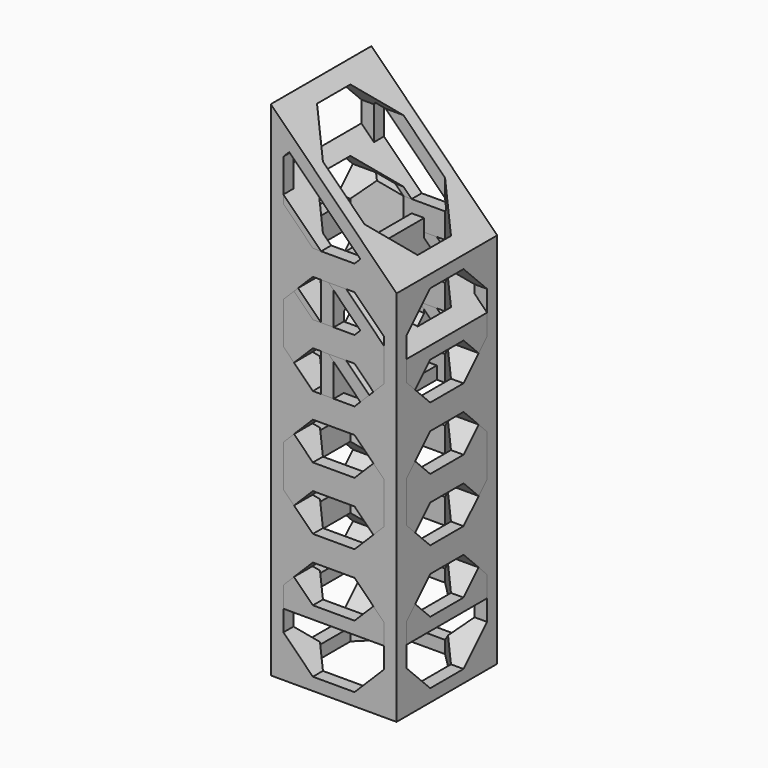
from build123d import *

# Parameters (mm, degrees)
F0_W      = 10
F0_H      = 10
F1_DEPTH  = 5
F3_DEPTH  = 10
F5_DEPTH  = 10
F7_DEPTH  = 10
F8_W      = 10
F8_H      = 20
F9_DEPTH  = 5
F11_DEPTH = 10
F13_DEPTH = 10
F15_DEPTH = 20
F17_DEPTH = 5
F19_DEPTH = 10
F21_DEPTH = 10
F23_DEPTH = 15
F25_DEPTH = 5
F27_DEPTH = 5
F29_DEPTH = 10
F31_DEPTH = 10
F33_DEPTH = 20
F35_DEPTH = 5
F37_DEPTH = 10
F39_DEPTH = 10
F41_DEPTH = 30
F43_DEPTH = 5
F45_DEPTH = 10
F47_DEPTH = 10
F49_DEPTH = 40


with BuildPart() as f1:
    # F0 (on Front) → F1 (new body, symmetric)
    with BuildSketch(Plane.XZ):
        Rectangle(F0_W, F0_H)
    extrude(amount=F1_DEPTH, both=True)

    # F2 (on face) → F3 (cut, through all)
    with BuildSketch(Plane.XZ.offset(5)):
        Polygon((4, 1.6568542495), (1.6568542495, 4), (-1.6568542495, 4), (-4, 1.6568542495), (-4, -1.6568542495), (-1.6568542495, -4), (1.6568542495, -4), (4, -1.6568542495), align=None)
    extrude(amount=-F3_DEPTH, mode=Mode.SUBTRACT)

    # F4 (on face) → F5 (cut, through all)
    with BuildSketch(Plane.YZ.offset(5)):
        Polygon((-1.6568542495, 4), (-4, 1.6568542495), (-4, -1.6568542495), (-1.6568542495, -4), (1.6568542495, -4), (4, -1.6568542495), (4, 1.6568542495), (1.6568542495, 4), align=None)
    extrude(amount=-F5_DEPTH, mode=Mode.SUBTRACT)

    # F6 (on face) → F7 (cut, through all)
    with BuildSketch(Plane.XY.offset(5)):
        Polygon((-1.6568542495, 4), (-4, 1.6568542495), (-4, -1.6568542495), (-1.6568542495, -4), (1.6568542495, -4), (4, -1.6568542495), (4, 1.6568542495), (1.6568542495, 4), align=None)
    extrude(amount=-F7_DEPTH, mode=Mode.SUBTRACT)


with BuildPart() as f9:
    # F8 (on Front) → F9 (new body, symmetric)
    with BuildSketch(Plane.XZ):
        Rectangle(F8_W, F8_H)
    extrude(amount=F9_DEPTH, both=True)

    # F10 (on face) → F11 (cut, through all)
    with BuildSketch(Plane.XZ.offset(5)):
        Polygon((4, 3.3431457505), (4, 6.6568542495), (1.6568542495, 9), (-1.6568542495, 9), (-4, 6.6568542495), (-4, 3.3431457505), (-1.6568542495, 1), (1.6568542495, 1), align=None)
        Polygon((4, -6.6568542495), (4, -3.3431457505), (1.6568542495, -1), (-1.6568542495, -1), (-4, -3.3431457505), (-4, -6.6568542495), (-1.6568542495, -9), (1.6568542495, -9), align=None)
    extrude(amount=-F11_DEPTH, mode=Mode.SUBTRACT)

    # F12 (on face) → F13 (cut, through all)
    with BuildSketch(Plane.YZ.offset(5)):
        Polygon((4, 3.3431457505), (4, 6.6568542495), (1.6568542495, 9), (-1.6568542495, 9), (-4, 6.6568542495), (-4, 3.3431457505), (-1.6568542495, 1), (1.6568542495, 1), align=None)
        Polygon((4, -6.6568542495), (4, -3.3431457505), (1.6568542495, -1), (-1.6568542495, -1), (-4, -3.3431457505), (-4, -6.6568542495), (-1.6568542495, -9), (1.6568542495, -9), align=None)
    extrude(amount=-F13_DEPTH, mode=Mode.SUBTRACT)

    # F14 (on face) → F15 (cut, through all)
    with BuildSketch(Plane.XY.offset(10)):
        Polygon((-1.6568542495, 4), (-4, 1.6568542495), (-4, -1.6568542495), (-1.6568542495, -4), (1.6568542495, -4), (4, -1.6568542495), (4, 1.6568542495), (1.6568542495, 4), align=None)
    extrude(amount=-F15_DEPTH, mode=Mode.SUBTRACT)


with BuildPart() as f17:
    # F16 (on Front) → F17 (new body, symmetric)
    with BuildSketch(Plane.XZ):
        Polygon((0, 10), (-5, 10), (-5, -10), (5, -10), (5, 0), (0, 0), align=None)
    extrude(amount=F17_DEPTH, both=True)

    # F18 (on face) → F19 (cut, through all)
    with BuildSketch(Plane.XZ.offset(5)):
        Polygon((4, -6.6568542495), (4, -3.3431457505), (1.6568542495, -1), (-1.6568542495, -1), (-4, -3.3431457505), (-4, -6.6568542495), (-1.6568542495, -9), (1.6568542495, -9), align=None)
        Polygon((-4, 3.3431457505), (-1.6568542495, 1), (-1, 1), (-1, 9), (-1.6568542495, 9), (-4, 6.6568542495), align=None)
    extrude(amount=-F19_DEPTH, mode=Mode.SUBTRACT)

    # F20 (on face) → F21 (cut, through all)
    with BuildSketch(Plane.YZ.offset(5)):
        Polygon((4, 3.3431457505), (4, 6.6568542495), (1.6568542495, 9), (-1.6568542495, 9), (-4, 6.6568542495), (-4, 3.3431457505), (-1.6568542495, 1), (1.6568542495, 1), align=None)
        Polygon((4, -6.6568542495), (4, -3.3431457505), (1.6568542495, -1), (-1.6568542495, -1), (-4, -3.3431457505), (-4, -6.6568542495), (-1.6568542495, -9), (1.6568542495, -9), align=None)
    extrude(amount=-F21_DEPTH, mode=Mode.SUBTRACT)

    # F22 (on face) → F23 (cut)
    with BuildSketch(Plane.XY.offset(10)):
        Polygon((-4, 1.6568542495), (-4, -1.6568542495), (-1.6568542495, -4), (-1, -4), (-1, 4), (-1.6568542495, 4), align=None)
        Polygon((1.6568542495, 4), (1, 4), (1, -4), (1.6568542495, -4), (4, -1.6568542495), (4, 1.6568542495), align=None)
    extrude(amount=-F23_DEPTH, mode=Mode.SUBTRACT)

    # F24 (on face) → F25 (cut)
    with BuildSketch(Plane(origin=(0, 0, -10), x_dir=(1, 0, 0), z_dir=(0, 0, -1))):
        Polygon((4, -1.6568542495), (4, 1.6568542495), (1.6568542495, 4), (-1.6568542495, 4), (-4, 1.6568542495), (-4, -1.6568542495), (-1.6568542495, -4), (1.6568542495, -4), align=None)
    extrude(amount=-F25_DEPTH, mode=Mode.SUBTRACT)


with BuildPart() as f27:
    # F26 (on Front) → F27 (new body, symmetric)
    with BuildSketch(Plane.XZ):
        Polygon((-5, -10), (5, -10), (5, 0), (-5, 10), align=None)
    extrude(amount=F27_DEPTH, both=True)

    # F28 (on face) → F29 (cut, through all)
    with BuildSketch(Plane.XZ.offset(5)):
        Polygon((4, -6.6568542495), (4, -3.3431457505), (1.6568542495, -1), (-1.6568542495, -1), (-4, -3.3431457505), (-4, -6.6568542495), (-1.6568542495, -9), (1.6568542495, -9), align=None)
        Polygon((-1.6568542495, 1), (1.6568542495, 1), (2.1213203436, 1.4644660941), (-3.5355339059, 7.1213203436), (-4, 6.6568542495), (-4, 3.3431457505), align=None)
    extrude(amount=-F29_DEPTH, mode=Mode.SUBTRACT)

    # F30 (on face) → F31 (cut, through all)
    with BuildSketch(Plane.YZ.offset(5)):
        Polygon((4, -6.6568542495), (4, -3.3431457505), (1.6568542495, -1), (-1.6568542495, -1), (-4, -3.3431457505), (-4, -6.6568542495), (-1.6568542495, -9), (1.6568542495, -9), align=None)
        Polygon((4, 3.3431457505), (4, 6.6568542495), (1.6568542495, 9), (-1.6568542495, 9), (-4, 6.6568542495), (-4, 3.3431457505), (-1.6568542495, 1), (1.6568542495, 1), align=None)
    extrude(amount=-F31_DEPTH, mode=Mode.SUBTRACT)

    # F32 (on face) → F33 (cut)
    with BuildSketch(Plane(origin=(0, 0, -10), x_dir=(1, 0, 0), z_dir=(0, 0, -1))):
        Polygon((-4, 1.6568542495), (-4, -1.6568542495), (-1.6568542495, -4), (1.6568542495, -4), (4, -1.6568542495), (4, 1.6568542495), (1.6568542495, 4), (-1.6568542495, 4), align=None)
    extrude(amount=-F33_DEPTH, mode=Mode.SUBTRACT)


with BuildPart() as f35:
    # F34 (on Front) → F35 (new body, symmetric)
    with BuildSketch(Plane.XZ):
        Polygon((-5, 15), (-5, -15), (5, -15), (5, 5), align=None)
    extrude(amount=F35_DEPTH, both=True)

    # F36 (on face) → F37 (cut, through all)
    with BuildSketch(Plane.XZ.offset(5)):
        Polygon((-4, 1.6568542495), (-4, -1.6568542495), (-1.6568542495, -4), (1.6568542495, -4), (4, -1.6568542495), (4, 1.6568542495), (1.6568542495, 4), (-1.6568542495, 4), align=None)
        Polygon((-4, -8.3431457505), (-4, -11.6568542495), (-1.6568542495, -14), (1.6568542495, -14), (4, -11.6568542495), (4, -8.3431457505), (1.6568542495, -6), (-1.6568542495, -6), align=None)
        Polygon((-4, 11.6568542495), (-4, 8.3431457505), (-1.6568542495, 6), (1.6568542495, 6), (2.1213203436, 6.4644660941), (-3.5355339059, 12.1213203436), align=None)
    extrude(amount=-F37_DEPTH, mode=Mode.SUBTRACT)

    # F38 (on face) → F39 (cut, through all)
    with BuildSketch(Plane.YZ.offset(5)):
        Polygon((4, -11.6568542495), (4, -8.3431457505), (1.6568542495, -6), (-1.6568542495, -6), (-4, -8.3431457505), (-4, -11.6568542495), (-1.6568542495, -14), (1.6568542495, -14), align=None)
        Polygon((4, -1.6568542495), (4, 1.6568542495), (1.6568542495, 4), (-1.6568542495, 4), (-4, 1.6568542495), (-4, -1.6568542495), (-1.6568542495, -4), (1.6568542495, -4), align=None)
        Polygon((4, 8.3431457505), (4, 11.6568542495), (1.6568542495, 14), (-1.6568542495, 14), (-4, 11.6568542495), (-4, 8.3431457505), (-1.6568542495, 6), (1.6568542495, 6), align=None)
    extrude(amount=-F39_DEPTH, mode=Mode.SUBTRACT)

    # F40 (on face) → F41 (cut)
    with BuildSketch(Plane(origin=(0, 0, -15), x_dir=(1, 0, 0), z_dir=(0, 0, -1))):
        Polygon((4, -1.6568542495), (4, 1.6568542495), (1.6568542495, 4), (-1.6568542495, 4), (-4, 1.6568542495), (-4, -1.6568542495), (-1.6568542495, -4), (1.6568542495, -4), align=None)
    extrude(amount=-F41_DEPTH, mode=Mode.SUBTRACT)


with BuildPart() as f43:
    # F42 (on Front) → F43 (new body, symmetric)
    with BuildSketch(Plane.XZ):
        Polygon((-5, 20), (-5, -20), (5, -20), (5, 10), align=None)
    extrude(amount=F43_DEPTH, both=True)

    # F44 (on face) → F45 (cut, through all)
    with BuildSketch(Plane.XZ.offset(5)):
        Polygon((-1.6568542495, 11), (1.6568542495, 11), (2.1213203436, 11.4644660941), (-3.5355339059, 17.1213203436), (-4, 16.6568542495), (-4, 13.3431457505), align=None)
        Polygon((4, 3.3431457505), (4, 6.6568542495), (1.6568542495, 9), (-1.6568542495, 9), (-4, 6.6568542495), (-4, 3.3431457505), (-1.6568542495, 1), (1.6568542495, 1), align=None)
        Polygon((4, -6.6568542495), (4, -3.3431457505), (1.6568542495, -1), (-1.6568542495, -1), (-4, -3.3431457505), (-4, -6.6568542495), (-1.6568542495, -9), (1.6568542495, -9), align=None)
        Polygon((4, -16.6568542495), (4, -13.3431457505), (1.6568542495, -11), (-1.6568542495, -11), (-4, -13.3431457505), (-4, -16.6568542495), (-1.6568542495, -19), (1.6568542495, -19), align=None)
    extrude(amount=-F45_DEPTH, mode=Mode.SUBTRACT)

    # F46 (on face) → F47 (cut, through all)
    with BuildSketch(Plane.YZ.offset(5)):
        Polygon((4, 13.3431457505), (4, 16.6568542495), (1.6568542495, 19), (-1.6568542495, 19), (-4, 16.6568542495), (-4, 13.3431457505), (-1.6568542495, 11), (1.6568542495, 11), align=None)
        Polygon((4, 3.3431457505), (4, 6.6568542495), (1.6568542495, 9), (-1.6568542495, 9), (-4, 6.6568542495), (-4, 3.3431457505), (-1.6568542495, 1), (1.6568542495, 1), align=None)
        Polygon((4, -6.6568542495), (4, -3.3431457505), (1.6568542495, -1), (-1.6568542495, -1), (-4, -3.3431457505), (-4, -6.6568542495), (-1.6568542495, -9), (1.6568542495, -9), align=None)
        Polygon((4, -16.6568542495), (4, -13.3431457505), (1.6568542495, -11), (-1.6568542495, -11), (-4, -13.3431457505), (-4, -16.6568542495), (-1.6568542495, -19), (1.6568542495, -19), align=None)
    extrude(amount=-F47_DEPTH, mode=Mode.SUBTRACT)

    # F48 (on face) → F49 (cut)
    with BuildSketch(Plane(origin=(0, 0, -20), x_dir=(1, 0, 0), z_dir=(0, 0, -1))):
        Polygon((4, -1.6568542495), (4, 1.6568542495), (1.6568542495, 4), (-1.6568542495, 4), (-4, 1.6568542495), (-4, -1.6568542495), (-1.6568542495, -4), (1.6568542495, -4), align=None)
    extrude(amount=-F49_DEPTH, mode=Mode.SUBTRACT)


solid = Compound([f1.part, f9.part, f17.part, f27.part, f35.part, f43.part])
